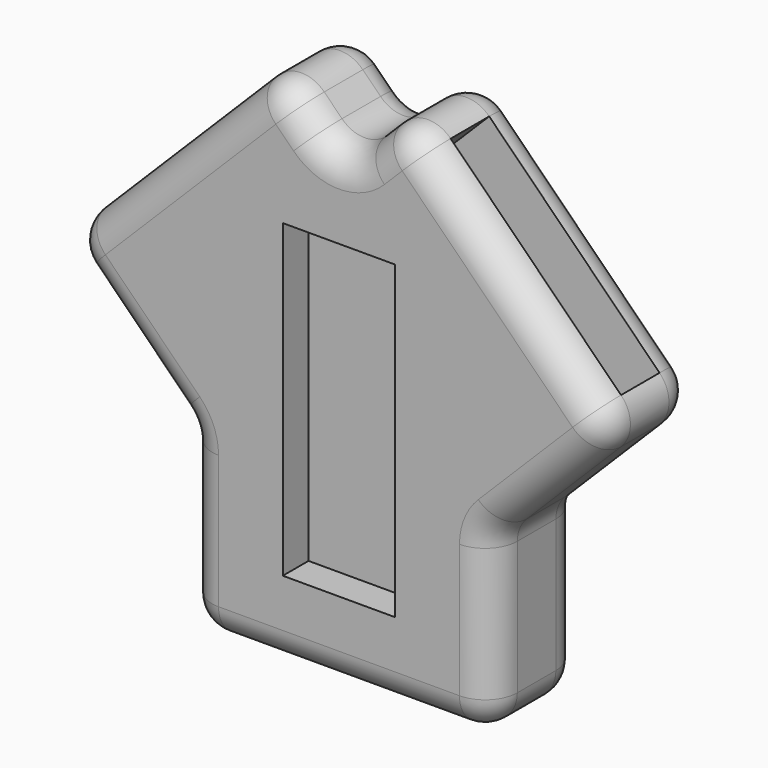
from build123d import *

# Parameters (mm, degrees)
F1_DEPTH  = 7
F2_W      = 15
F2_H      = 3
F3_DEPTH  = 25
F4_W      = 15
F4_H      = 3
F5_DEPTH  = 19.6
F6_W      = 3
F6_H      = 15
F7_DEPTH  = 21.3
F8_R      = 1.99999
F9_W      = 7
F9_H      = 19.3284271247
F10_DEPTH = 2


# Not quite as in the source:
# - a fillet or chamfer is up to 0.001 mm smaller than in the source, because OpenCascade refuses the exact size


with BuildPart() as f1:
    # F0 (on Front) → F1 (new body)
    with BuildSketch(Plane.XZ):
        Polygon((0, 9.5), (-9.5, 0), (9.5, 0), align=None)
        Polygon((9.5, 0), (-9.5, 0), (-9.5, -7.8700576851), (-9.5, -19), (9.5, -19), (9.5, -7.8700576851), align=None)
        Polygon((-9.5, -7.8700576851), (-9.5, 0), (0, 9.5), (-3.9350288425, 13.4350288425), (-17.3700576851, 0), align=None)
        Polygon((0, 9.5), (9.5, 0), (9.5, -7.8700576851), (17.3700576851, 0), (3.9350288425, 13.4350288425), align=None)
    extrude(amount=F1_DEPTH)

    # F2 (on face) → F3 (cut)
    with BuildSketch(Plane(origin=(0, 0, -19), x_dir=(1, 0, 0), z_dir=(0, 0, -1))):
        with Locations((0, 3.5)):
            Rectangle(F2_W, F2_H)
    extrude(amount=-F3_DEPTH, mode=Mode.SUBTRACT)

    # F4 (on face) → F5 (cut)
    with BuildSketch(Plane(origin=(8.6850288425, 0, 8.6850288425), x_dir=(0.7071067812, 0, -0.7071067812), z_dir=(0.7071067812, 0, 0.7071067812))):
        with Locations((2.7824855787, -3.5)):
            Rectangle(F4_W, F4_H)
    extrude(amount=-F5_DEPTH, mode=Mode.SUBTRACT)

    # F6 (on face) → F7 (cut)
    with BuildSketch(Plane(origin=(-8.6850288425, 0, 8.6850288425), x_dir=(0, -1, 0), z_dir=(-0.7071067812, 0, 0.7071067812))):
        with Locations((3.5, -2.7824855787)):
            Rectangle(F6_W, F6_H)
    extrude(amount=-F7_DEPTH, mode=Mode.SUBTRACT)

    # F8 (radius 2 in the source; OpenCascade refuses exactly that, so slightly less here)
    f8_edges = [f1.edges().sort_by_distance(p)[0] for p in [
        (-9.5, -7, -13.435029),
        (-13.435029, -7, -3.935029),
        (-13.435029, 0, -3.935029),
        (-9.5, 0, -13.435029),
        (0, -7, -19),
        (0, 0, -19),
        (-9.5, -3.5, -19),
        (9.5, -3.5, -19),
        (9.5, -7, -13.435029),
        (9.5, 0, -13.435029),
        (13.435029, 0, -3.935029),
        (13.435029, -7, -3.935029),
        (17.370058, -3.5, 0),
        (10.652543, -7, 6.717514),
        (3.935029, -3.5, 13.435029),
        (10.652543, 0, 6.717514),
        (1.967514, 0, 11.467514),
        (-1.967514, 0, 11.467514),
        (-1.967514, -7, 11.467514),
        (1.967514, -7, 11.467514),
        (-10.652543, -7, 6.717514),
        (-3.935029, -3.5, 13.435029),
        (-10.652543, 0, 6.717514),
        (-17.370058, -3.5, 0),
        (0, -3.5, 9.5),
        (-9.5, -3.5, -7.870058),
        (9.5, -3.5, -7.870058),
    ]]
    fillet(f8_edges, radius=F8_R)

    # F9 (on face) → F10 (cut)
    with BuildSketch(Plane.XZ.offset(7)):
        with Locations((0, -4.3357864376)):
            Rectangle(F9_W, F9_H)
    extrude(amount=-F10_DEPTH, mode=Mode.SUBTRACT)


solid = f1.part
